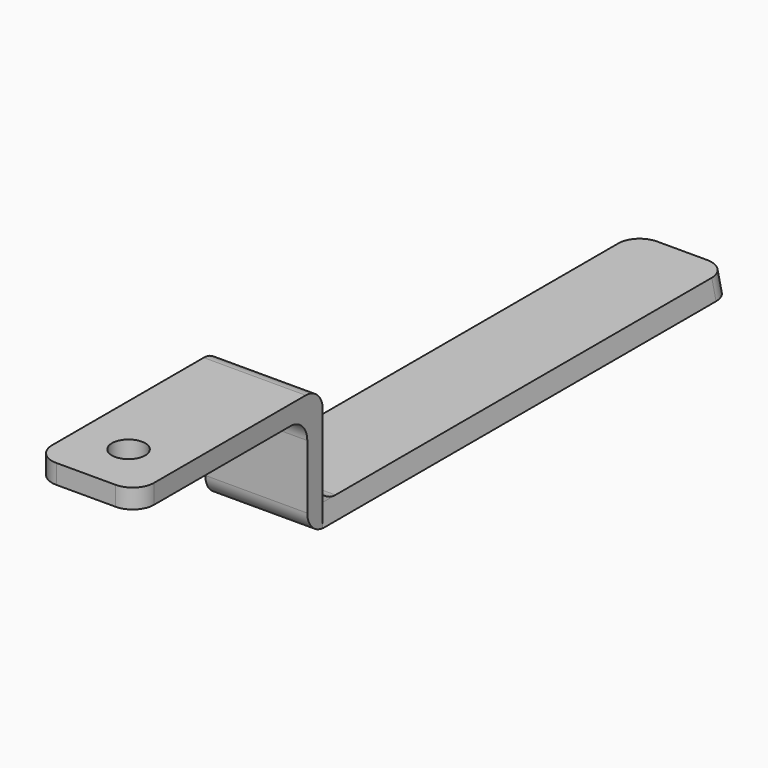
from build123d import *

# Parameters (mm, degrees)
F1_DEPTH      = 127
F2_W          = 24.3321505244
F2_H          = 4.6101
F3_DEPTH      = 25.4
F3_DEPTH_BACK = 4.6101
F4_W          = 24.3321505244
F4_H          = 4.6101
F5_DEPTH      = 50.8
F6_T1_DEPTH   = 24.3321505244
F6_T6_DEPTH   = 47.6747505244
F6_T9_DEPTH   = 49.7321505244
F6_T11_DEPTH  = 30.0101
F6_T13_DEPTH  = 30.1234781359
F6_T15_DEPTH  = 30.1234781359
F8_D          = 7.9375
F8_DEPTH      = 19.05
F8_TIP        = 2.3846655818


# Not quite as in the source:
# - a fillet or chamfer that OpenCascade refuses, or shapes differently, is made with other operations: its cross-section is extruded or revolved along the edge and cut away or added


with BuildPart() as f1:
    # F0 (on Front) → F1 (new body)
    with BuildSketch(Plane.XZ):
        Polygon((1.8483747378, 4.6101), (0.8196747378, 0), (25.1518252622, 0), (24.1231252622, 4.6101), align=None)
    extrude(amount=F1_DEPTH)

    # F2 (on face) → F3 (join, two sides)
    with BuildSketch(Plane.XY.offset(4.6101)) as f3_sk:
        with Locations((12.98575, -124.69495)):
            Rectangle(F2_W, F2_H)
    extrude(amount=F3_DEPTH)
    extrude(f3_sk.sketch, amount=-F3_DEPTH_BACK)

    # F4 (on face) → F5 (join)
    with BuildSketch(Plane.XZ.offset(127)):
        with Locations((12.98575, 27.70505)):
            Rectangle(F4_W, F4_H)
    extrude(amount=F5_DEPTH)

    # F6: fillet of radius 5.08 on 8 edges, made by hand

    # F6_s2 → F6_t1 (join)
    with BuildSketch(Plane.YZ.offset(0.8196747378)):
        with BuildLine():
            ThreePointArc((-132.08, 25.4), (-128.4878975516, 23.9121024484), (-127, 20.32))
            Line((-127, 20.32), (-127, 25.4))
            Line((-127, 25.4), (-132.08, 25.4))
        make_face()
    extrude(amount=F6_T1_DEPTH)


with BuildPart() as f6_tool4:
    # F6_s5 → F6_t6 (new body)
    with BuildSketch(Plane.YZ.offset(36.8231252622)):
        with BuildLine():
            ThreePointArc((-117.3099, 4.6101), (-120.9020024484, 6.0979975516), (-122.3899, 9.6901))
            Line((-122.3899, 9.6901), (-122.3899, 4.6101))
            Line((-122.3899, 4.6101), (-117.3099, 4.6101))
        make_face()
    extrude(amount=-F6_T6_DEPTH)

    split(bisect_by=Plane(origin=(0.780797517, 0, -0.1742275451), x_dir=(0, 1, 0), z_dir=(0.9759968962, 0, -0.2177844314)), keep=Keep.TOP)

    split(bisect_by=Plane(origin=(23.9588727172, 0, 5.3461947386), x_dir=(0, 1, 0), z_dir=(-0.9759968962, 0, -0.2177844314)), keep=Keep.TOP)


with BuildPart() as f1_1:
    add(f1.part)

    # F6_t3: union F6_tool4
    add(f6_tool4.part)

    # F6_s10 → F6_t9 (cut)
    with BuildSketch(Plane.YZ.offset(-11.8803252622)):
        with BuildLine():
            ThreePointArc((-127.4699, 30.0101), (-123.8777975516, 28.5222024484), (-122.3899, 24.9301))
            Line((-122.3899, 24.9301), (-122.3899, 30.0101))
            Line((-122.3899, 30.0101), (-127.4699, 30.0101))
        make_face()
        with BuildLine():
            ThreePointArc((-121.92, 0), (-125.5121024484, 1.4878975516), (-127, 5.08))
            Line((-127, 5.08), (-127, 0))
            Line((-127, 0), (-121.92, 0))
        make_face()
    extrude(amount=F6_T9_DEPTH, mode=Mode.SUBTRACT)

    # F6_s12 → F6_t11 (cut)
    with BuildSketch(Plane.XY.offset(12.7)):
        with BuildLine():
            ThreePointArc((5.8996747378, -177.8), (2.3075722894, -176.3121024484), (0.8196747378, -172.72))
            Line((0.8196747378, -172.72), (0.8196747378, -177.8))
            Line((0.8196747378, -177.8), (5.8996747378, -177.8))
        make_face()
        with BuildLine():
            ThreePointArc((25.1518252622, -172.72), (23.6639277106, -176.3121024484), (20.0718252622, -177.8))
            Line((20.0718252622, -177.8), (25.1518252622, -177.8))
            Line((25.1518252622, -177.8), (25.1518252622, -172.72))
        make_face()
    extrude(amount=F6_T11_DEPTH, mode=Mode.SUBTRACT)

    # F6_s14 → F6_t13 (cut)
    with BuildSketch(Plane(origin=(3.8334394995, 0, 17.1794881272), x_dir=(0, 1, 0), z_dir=(-0.2177844314, 0, -0.9759968962))):
        with BuildLine():
            ThreePointArc((-5.08, 0.8), (-1.4878975516, 2.2878975516), (0, 5.88))
            Line((0, 5.88), (0, 0.8))
            Line((0, 0.8), (-5.08, 0.8))
        make_face()
    extrude(amount=F6_T13_DEPTH, mode=Mode.SUBTRACT)

    # F6_s16 → F6_t15 (cut)
    with BuildSketch(Plane(origin=(3.9588148236, 0, -17.7413553206), x_dir=(0, 1, 0), z_dir=(-0.2177844314, 0, 0.9759968962))):
        with BuildLine():
            ThreePointArc((-5.08, -24.5481033904), (-1.4878975516, -23.0602058388), (0, -19.4681033904))
            Line((0, -19.4681033904), (0, -24.5481033904))
            Line((0, -24.5481033904), (-5.08, -24.5481033904))
        make_face()
    extrude(amount=F6_T15_DEPTH, mode=Mode.SUBTRACT)

    # F8
    with Locations(Plane.XY.offset(30.0101)):
        with Locations((12.98575, -165.1)):
            Hole(F8_D / 2, depth=F8_DEPTH)
            with Locations((0, 0, -(F8_DEPTH + F8_TIP / 2))):  # 118° drill point
                Cone(0, F8_D / 2, F8_TIP, mode=Mode.SUBTRACT)


solid = f1_1.part
